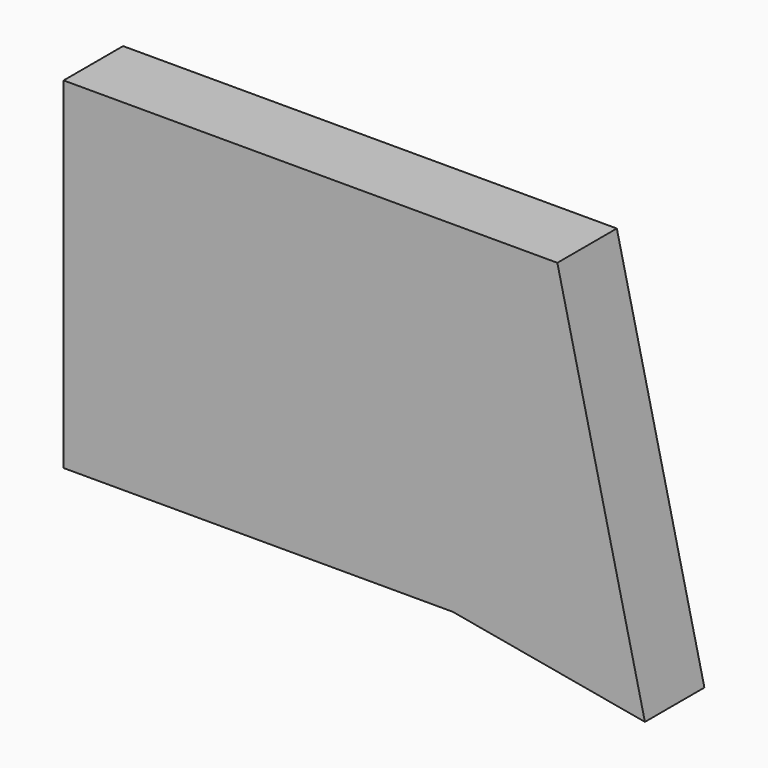
from build123d import *

# Parameters (mm, degrees)
F3_DEPTH = 25.4


# Not quite as in the source:
# - the program builds the solid bodies; features that only make, move or delete a surface that nothing else refers to are left out


with BuildPart() as f3:
    # F2 (on Front) → F3 (new body)
    with BuildSketch(Plane.XZ):
        Polygon((157.005161047, -81.5721079707), (289.9789810181, -81.5721079707), (355.6255698204, -93.3439582586), (325.7018923759, 35.0206755102), (157.005161047, 35.0206755102), align=None)
    extrude(amount=F3_DEPTH)


solid = f3.part
